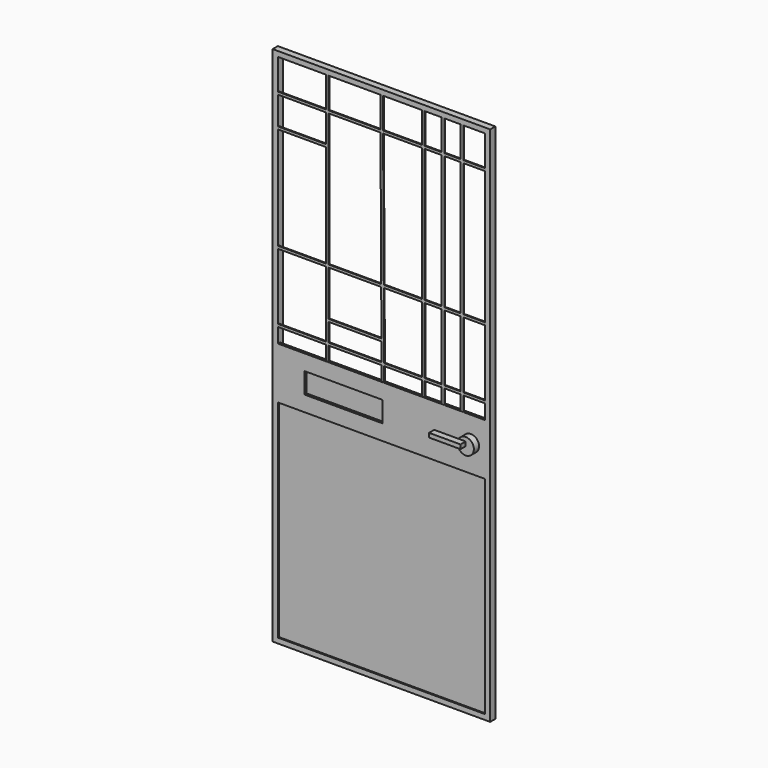
from build123d import *

# Parameters (mm, degrees)
F0_W          = 840
F0_H          = 2015
F1_DEPTH      = 20
F1_DEPTH_BACK = 5
F0_W_2        = 800
F0_H_2        = 800
F2_DEPTH      = 5
F3_DEPTH      = 5
F3_DEPTH_BACK = 5
F0_W_3        = 66.3491392136
F0_H_3        = 255.5529880524
F0_W_4        = 63.4402632713
F0_H_4        = 514.2461061478
F4_DEPTH      = 4
F5_W          = 300
F5_H          = 80
F6_DEPTH      = 25
F7_R          = 31.4858803301
F8_DEPTH      = 25
F10_DEPTH     = 25
F11_W         = 324.000005722
F11_H         = 104.000005722
F11_W_2       = 300
F11_H_2       = 80
F12_DEPTH     = 5


# Not quite as in the source:
# - a feature names something its author has since deleted; it is built from what else it names


with BuildPart() as f1:
    # F0 (on Front) → F1 (new body, two sides)
    with BuildSketch(Plane.XZ) as f1_sk:
        with Locations((420, 1007.5)):
            Rectangle(F0_W, F0_H)
        Polygon((20, 1875.9479618073), (20, 1995), (204.9973701685, 1995), (214.9973701685, 1995), (415, 1995), (425, 1995), (575.6211781502, 1995), (585.6211781502, 1995), (651.9703173637, 1995), (661.9703173637, 1995), (725.4105806351, 1995), (735.4105806351, 1995), (820, 1995), (820, 1875.9479618073), (820, 1865.9479618073), (820, 1351.7018556595), (820, 1341.7018556595), (820, 1086.1488676071), (820, 1076.1488676071), (820, 1020), (820, 820), (820, 20), (20, 20), (20, 820), (20, 1020), (20, 1076.1488676071), (20, 1086.1488676071), (20, 1341.7018556595), (20, 1351.7018556595), (20, 1747.877240181), (20, 1757.877240181), (20, 1865.9479618073), align=None, mode=Mode.SUBTRACT)
    extrude(amount=-F1_DEPTH)
    extrude(f1_sk.sketch, amount=F1_DEPTH_BACK)

    # F0 (on Front) → F2 (join)
    with BuildSketch(Plane.XZ):
        with Locations((420, 420)):
            Rectangle(F0_W_2, F0_H_2)
    extrude(amount=-F2_DEPTH)

    # F0 (on Front) → F3 (join, two sides)
    with BuildSketch(Plane.XZ) as f3_sk:
        Polygon((204.9973701685, 1020), (20, 1020), (20, 820), (820, 820), (820, 1020), (735.4105806351, 1020), (725.4105806351, 1020), (661.9703173637, 1020), (651.9703173637, 1020), (585.6211781502, 1020), (575.6211781502, 1020), (430, 1020), (420, 1020), (214.9973701685, 1020), align=None)
    extrude(amount=F3_DEPTH)
    extrude(f3_sk.sketch, amount=-F3_DEPTH_BACK)

    # F0 (on Front) → F4 (join)
    with BuildSketch(Plane.XZ):
        Polygon((214.9973701685, 1995), (204.9973701685, 1995), (204.9973701685, 1875.9479618073), (20, 1875.9479618073), (20, 1865.9479618073), (204.9973701685, 1865.9479618073), (204.9973701685, 1757.877240181), (20, 1757.877240181), (20, 1747.877240181), (204.9973701685, 1747.877240181), (204.9973701685, 1351.7018556595), (20, 1351.7018556595), (20, 1341.7018556595), (204.9973701685, 1341.7018556595), (204.9973701685, 1086.1488676071), (20, 1086.1488676071), (20, 1076.1488676071), (204.9973701685, 1076.1488676071), (204.9973701685, 1020), (214.9973701685, 1020), (214.9973701685, 1076.1488676071), (419.7120570892, 1076.1488676071), (420, 1020), (430, 1020), (429.7120570892, 1076.1488676071), (575.6211781502, 1076.1488676071), (575.6211781502, 1020), (585.6211781502, 1020), (585.6211781502, 1076.1488676071), (651.9703173637, 1076.1488676071), (651.9703173637, 1020), (661.9703173637, 1020), (661.9703173637, 1076.1488676071), (725.4105806351, 1076.1488676071), (725.4105806351, 1020), (735.4105806351, 1020), (735.4105806351, 1076.1488676071), (820, 1076.1488676071), (820, 1086.1488676071), (735.4105806351, 1086.1488676071), (735.4105806351, 1341.7018556595), (820, 1341.7018556595), (820, 1351.7018556595), (735.4105806351, 1351.7018556595), (735.4105806351, 1865.9479618073), (820, 1865.9479618073), (820, 1875.9479618073), (735.4105806351, 1875.9479618073), (735.4105806351, 1995), (725.4105806351, 1995), (725.4105806351, 1875.9479618073), (661.9703173637, 1875.9479618073), (661.9703173637, 1995), (651.9703173637, 1995), (651.9703173637, 1875.9479618073), (585.6211781502, 1875.9479618073), (585.6211781502, 1995), (575.6211781502, 1995), (575.6211781502, 1875.9479618073), (425.6105232728, 1875.9479618073), (425, 1995), (415, 1995), (415.6105232728, 1875.9479618073), (214.9973701685, 1875.9479618073), align=None)
        Polygon((214.9973701685, 1086.1488676071), (214.9973701685, 1156.8437051624), (419.2982374094, 1156.8437051624), (419.6607750379, 1086.1488676071), align=None, mode=Mode.SUBTRACT)
        Polygon((419.2469553581, 1166.8437051624), (214.9973701685, 1166.8437051624), (214.9973701685, 1341.7018556595), (418.3502468941, 1341.7018556595), align=None, mode=Mode.SUBTRACT)
        Polygon((418.2989648428, 1351.7018556595), (214.9973701685, 1351.7018556595), (214.9973701685, 1865.9479618073), (415.6618053241, 1865.9479618073), align=None, mode=Mode.SUBTRACT)
        Polygon((575.6211781502, 1086.1488676071), (429.6607750379, 1086.1488676071), (428.3502468941, 1341.7018556595), (575.6211781502, 1341.7018556595), align=None, mode=Mode.SUBTRACT)
        with Locations((618.795747757, 1213.9253616333)):
            Rectangle(F0_W_3, F0_H_3, mode=Mode.SUBTRACT)
        with Locations((693.6904489994, 1213.9253616333)):
            Rectangle(F0_W_4, F0_H_3, mode=Mode.SUBTRACT)
        Polygon((428.2989648428, 1351.7018556595), (425.6618053241, 1865.9479618073), (575.6211781502, 1865.9479618073), (575.6211781502, 1351.7018556595), align=None, mode=Mode.SUBTRACT)
        with Locations((618.795747757, 1608.8249087334)):
            Rectangle(F0_W_3, F0_H_4, mode=Mode.SUBTRACT)
        with Locations((693.6904489994, 1608.8249087334)):
            Rectangle(F0_W_4, F0_H_4, mode=Mode.SUBTRACT)
    extrude(amount=F4_DEPTH)

    # F5 (on face) → F6 (cut)
    with BuildSketch(Plane.XZ.offset(5)):
        with Locations((273.4116579701, 920)):
            Rectangle(F5_W, F5_H)
    extrude(amount=-F6_DEPTH, mode=Mode.SUBTRACT)

    # F7 (on face) → F8 (join)
    with BuildSketch(Plane.XZ.offset(5)):
        with Locations((765.6806707382, 923.5473275185)):
            Circle(F7_R)
    extrude(amount=F8_DEPTH)

    # F9 (on face) → F10 (join)
    with BuildSketch(Plane.XZ.offset(30)):
        with BuildLine():
            Line((644.1951990128, 923.5473275185), (734.1947904082, 923.5473275185))
            ThreePointArc((734.1947904082, 923.5473275185), (735.3422931651, 931.9701243455), (738.701159971, 939.778983593))
            Line((738.701159971, 939.778983593), (644.1951990128, 939.778983593))
            Line((644.1951990128, 939.778983593), (644.1951990128, 923.5473275185))
        make_face()
        with BuildLine():
            Line((734.1947904082, 923.5473275185), (765.6806707382, 923.5473275185))
            Line((765.6806707382, 923.5473275185), (765.6806707382, 939.778983593))
            Line((765.6806707382, 939.778983593), (738.701159971, 939.778983593))
            ThreePointArc((738.701159971, 939.778983593), (735.3422931651, 931.9701243455), (734.1947904082, 923.5473275185))
        make_face()
    extrude(amount=F10_DEPTH)

    # F11 (on face) → F12 (join)
    with BuildSketch(Plane(origin=(0, 5, 0), x_dir=(-1, 0, 0), z_dir=(0, 1, 0))):
        with Locations((-273.4116579701, 920)):
            Rectangle(F11_W, F11_H)
        with Locations((-273.4116579701, 920)):
            Rectangle(F11_W_2, F11_H_2, mode=Mode.SUBTRACT)
        with Locations((-273.4116579701, 920)):
            Rectangle(F11_W_2, F11_H_2)
    extrude(amount=F12_DEPTH)


solid = f1.part
